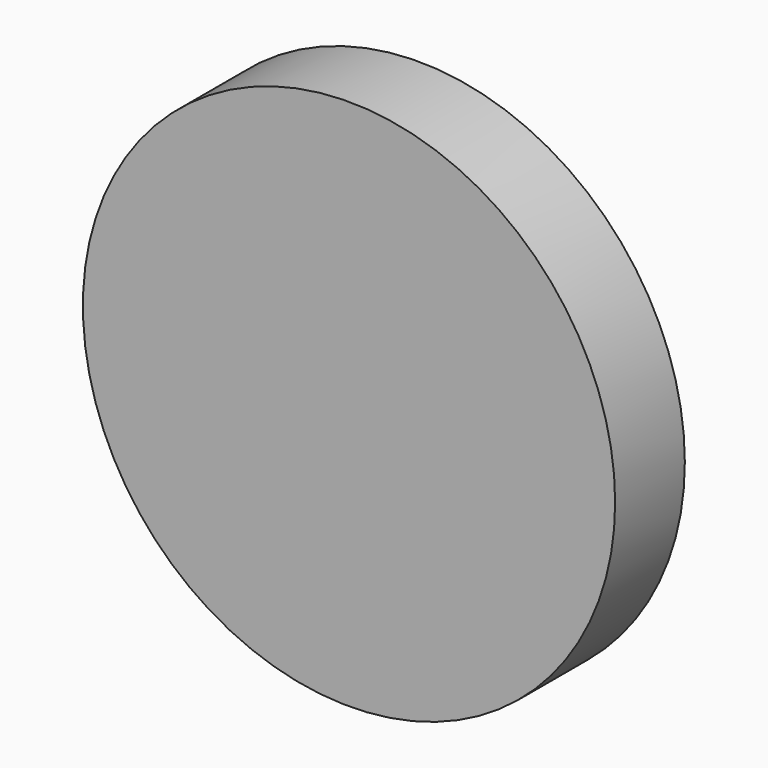
from build123d import *

# Parameters (mm, degrees)
F2_R          = 31.0373499358
F3_DEPTH      = 5.08
F3_DEPTH_BACK = 5.08


# Not quite as in the source:
# - the program builds the solid bodies; features that only make, move or delete a surface that nothing else refers to are left out


with BuildPart() as f3:
    # F2 (on Front) → F3 (new body, two sides)
    with BuildSketch(Plane.XZ) as f3_sk:
        Circle(F2_R)
    extrude(amount=F3_DEPTH)
    extrude(f3_sk.sketch, amount=-F3_DEPTH_BACK)


solid = f3.part
